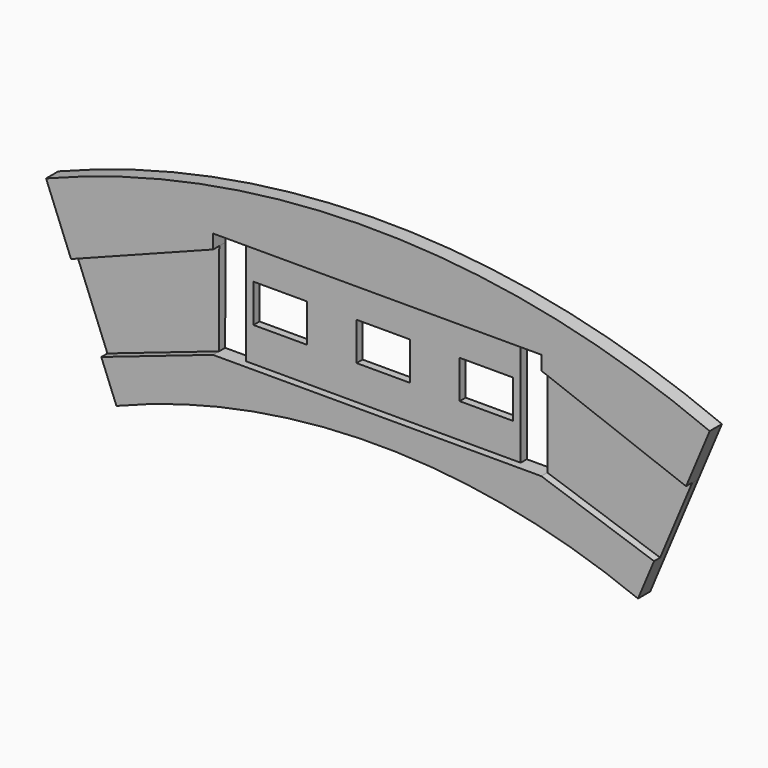
from build123d import *

# Parameters (mm, degrees)
F1_DEPTH = 2
F0_W     = 36
F0_H     = 14
F0_W_2   = 7
F0_H_2   = 5
F2_DEPTH = 1
F3_DEPTH = 2
F4_DEPTH = 1
F5_DEPTH = 1
F6_DEPTH = 2.001
F7_DEPTH = 2.001
F8_DEPTH = 1


# Not quite as in the source:
# - ends of sketch curves that miss each other by under 0.0002 mm in the source are joined


with BuildPart() as f1:
    # F0 (on Front) → F1 (new body)
    with BuildSketch(Plane.XZ):
        with BuildLine():
            Line((40.4628534786, 0), (43.5572046873, 7.3690142199))
            ThreePointArc((43.5572046873, 7.3690142199), (0.1833509298, 16.332060188), (-43.3610966095, 8.2383298181))
            Line((-43.3610966095, 8.2383298181), (-40.0939611875, 0))
            Line((-40.0939611875, 0), (-21.4795553588, 7.1586821743))
            Line((-21.4795553588, 7.1586821743), (-21.4764592054, 9.000000095))
            Line((-21.4764592054, 9.000000095), (-18, 9.000000095))
            Line((-18, 9.000000095), (18, 9.000000095))
            Line((18, 9.000000095), (21.5, 9.000000095))
            Line((21.5, 9.000000095), (21.5, 7.1586821743))
            Line((21.5, 7.1586821743), (40.4628534786, 0))
        make_face()
    extrude(amount=F1_DEPTH)

    # F0 (on Front) → F2 (join)
    with BuildSketch(Plane.XZ):
        Polygon((21.5, -4.999999905), (21.5, 7.1586821743), (21.5, 9.000000095), (18, 9.000000095), (18, -4.999999905), align=None)
        with Locations((0, 2.000000095)):
            Rectangle(F0_W, F0_H)
        with Locations((-13.5, 2.000000095)):
            Rectangle(F0_W_2, F0_H_2, mode=Mode.SUBTRACT)
        with Locations((0, 2.000000095)):
            Rectangle(F0_W_2, F0_H_2, mode=Mode.SUBTRACT)
        Polygon((17, 4.500000095), (17, -0.499999905), (15, -0.499999905), (10, -0.499999905), (10, 2.500000095), (10, 4.500000095), align=None, mode=Mode.SUBTRACT)
        Polygon((-21.4764592054, 9.000000095), (-21.4795553588, 7.1586821743), (-21.5, -4.9999801132), (-18, -4.999999905), (-18, 9.000000095), align=None)
    extrude(amount=F2_DEPTH)

    # F0 (on Front) → F3 (join)
    with BuildSketch(Plane.XZ):
        with BuildLine():
            Line((34.164145572, -15), (36.2637148742, -10))
            Line((36.2637148742, -10), (21.5, -4.999999905))
            Line((21.5, -4.999999905), (18, -4.999999905))
            Line((18, -4.999999905), (-18, -4.999999905))
            Line((-18, -4.999999905), (-21.5, -4.999999905))
            Line((-21.5, -4.999999905), (-36.1281871846, -10))
            Line((-36.1281871846, -10), (-34.1453001831, -15))
            ThreePointArc((-34.1453001831, -15), (0.0094226944, -8.3568901314), (34.164145572, -15))
        make_face()
    extrude(amount=F3_DEPTH)

    # F0 (on Front) → F4 (join)
    with BuildSketch(Plane.XZ):
        Polygon((36.2637148742, -10), (40.4628534786, 0), (21.5, 7.1586821743), (21.5, -4.999999905), align=None)
    extrude(amount=F4_DEPTH)

    # F0 (on Front) → F5 (join)
    with BuildSketch(Plane.XZ):
        Polygon((-21.4795553588, 7.1586821743), (-40.0939611875, 0), (-36.1281871846, -10), (-21.5, -4.999999905), align=None)
    extrude(amount=F5_DEPTH)

    # F0 (on Front) → F6 (cut, through all)
    with BuildSketch(Plane.XZ):
        Polygon((21.5, -4.999999905), (21.5, 7.1586821743), (21.5, 9.000000095), (18, 9.000000095), (18, -4.999999905), align=None)
    extrude(amount=F6_DEPTH, mode=Mode.SUBTRACT)

    # F0 (on Front) → F7 (cut, through all)
    with BuildSketch(Plane.XZ):
        Polygon((-21.4764592054, 9.000000095), (-21.4795553588, 7.1586821743), (-21.5, -4.9999801132), (-18, -4.999999905), (-18, 9.000000095), align=None)
    extrude(amount=F7_DEPTH, mode=Mode.SUBTRACT)

    # F0 (on Front) → F8 (join)
    with BuildSketch(Plane.XZ):
        with Locations((0, 2.000000095)):
            Rectangle(F0_W, F0_H)
        with Locations((-13.5, 2.000000095)):
            Rectangle(F0_W_2, F0_H_2, mode=Mode.SUBTRACT)
        with Locations((0, 2.000000095)):
            Rectangle(F0_W_2, F0_H_2, mode=Mode.SUBTRACT)
        Polygon((17, 4.500000095), (17, -0.499999905), (15, -0.499999905), (10, -0.499999905), (10, 2.500000095), (10, 4.500000095), align=None, mode=Mode.SUBTRACT)
    extrude(amount=F8_DEPTH)


solid = f1.part
